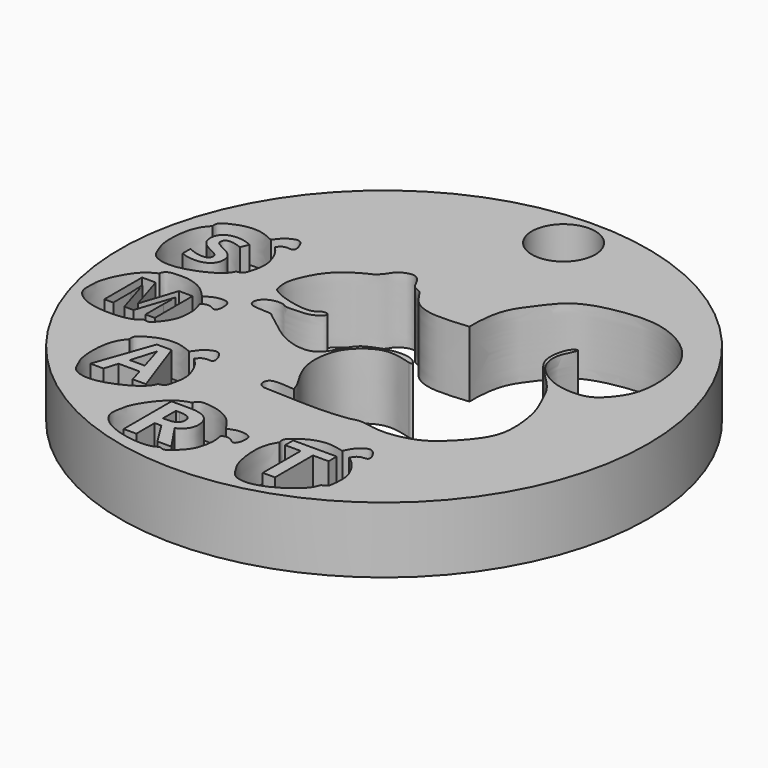
from build123d import *

# Parameters (mm, degrees)
F0_R           = 25.4
F1_DEPTH       = 6.35
F3_DEPTH       = 3.175
F4_TEXT_SIZE   = 6.6135069162
F4_TEXT_SIZE_2 = 6.365134491
F4_TEXT_SIZE_3 = 7.739350031
F4_TEXT_SIZE_4 = 8.0579310345
F4_TEXT_SIZE_5 = 7.7680943327
F5_DEPTH       = 3.175
F6_R           = 3.048
F7_DEPTH       = 25.4


# Not quite as in the source:
# - Text() gives the source's letters only with a copy of the font that has no kerning and outlines rounded to 1/6400 em; it was checked with that copy


with BuildPart() as f1:
    # F0 (on Top) → F1 (new body)
    with BuildSketch(Plane.XY):
        Circle(F0_R)
        with BuildLine():
            add(Edge.make_bspline(
                [(3.103984287, -0.8738507167), (3.2322647315, -0.8978823469), (3.5149160662, -0.9508333041), (3.1489052737, -0.3935869069), (2.1759216009, 0.01042191), (0.4678924032, -0.1717785151), (-0.6658792375, -0.6737219093), (-1.7045465622, -1.1078755571), (-2.5695800826, -2.8283012682), (-3.3167997934, -3.978649584), (-5.0026669085, -4.2655482317), (-7.292063398, -3.3539291003), (-8.8308556716, -1.9327427837), (-9.7776344556, -1.3804225536), (-9.9096110556, -1.0268847401), (-11.7269123051, -1.1581922681), (-12.2987806359, -0.6742192075), (-12.186278121, 0.0905562062), (-11.3044733094, 0.7354376931), (-10.1770359316, 0.7119397356), (-9.9059421857, 0.3673581843), (-8.4562468827, 0.44879459), (-7.5199595832, 0.5096907301), (-6.5266853491, 1.092838295), (-6.594417206, 1.6640416494), (-7.4144486566, 1.4846144189), (-7.7096041895, 1.0548830834), (-8.9475055661, 1.0261015402), (-10.6206031717, 1.4261002308), (-11.5516225248, 1.8097186625), (-11.9262345749, 2.0845401136), (-12.0926881209, 2.2066531237)],
                knots=[0, 0, 0, 0, 0.0184086765, 0.04056142, 0.0760871843, 0.1209751136, 0.1592656487, 0.1947406005, 0.2417782506, 0.2813138073, 0.3236254209, 0.3775272699, 0.42833216, 0.4622779251, 0.4810085106, 0.5258803693, 0.5538009145, 0.5810631125, 0.6164897777, 0.6512938544, 0.6727879582, 0.7125289418, 0.7482314257, 0.7830455257, 0.8029526961, 0.8310756273, 0.8553552773, 0.8920195713, 0.9381311083, 0.9725094363, 1, 1, 1, 1], degree=3))
            add(Edge.make_bspline(
                [(-12.0926881209, 2.2066531237), (-12.1940696834, 2.6175798085), (-12.4176238462, 3.5237048342), (-11.7188787033, 5.3710118016), (-10.5601116678, 7.2426050922), (-8.4458315601, 8.4856568685), (-7.8733042, 8.650989017), (-7.19697809, 9.3700944594), (-6.9202423533, 10.0770039736), (-5.3336173542, 10.8016234373), (-4.5255374898, 9.5922548337), (-4.2877600091, 8.857299522), (-3.3906737996, 8.7893316439), (-2.7399658464, 7.2252450905), (-0.7680652696, 6.1582634822), (1.620715387, 6.3925439066), (2.9963927809, 6.5274639055)],
                knots=[0, 0, 0, 0, 0.0677915818, 0.1494856652, 0.2403248537, 0.3309571532, 0.3772706487, 0.4332906216, 0.4864872395, 0.5575025948, 0.6239020411, 0.6741953722, 0.7244037027, 0.7978595843, 0.8835891443, 1, 1, 1, 1], degree=3))
            add(Edge.make_bspline(
                [(2.9963927809, 6.5274639055), (2.9876517934, 6.8087234454), (2.9646580281, 7.5485958891), (3.2208507353, 10.2567825473), (4.8072550972, 12.248326722), (6.4649635254, 14.6254966411), (10.2089734272, 15.6611927232), (14.460945516, 15.9289527113), (18.5488481139, 13.4786584252), (19.8526536032, 9.7353067267), (19.8012884144, 6.002184071), (18.3256681545, 4.0448117291), (17.1799807769, 3.0665154622), (15.2183525329, 2.921829898), (13.2866030879, 3.370569802), (11.2108415273, 4.8912140214), (10.9518605827, 6.9579767834), (11.7126375257, 8.1676137563), (11.835203024, 8.7609334617), (11.0376890387, 8.3226443822), (10.6454263926, 6.4262151181), (11.1367654893, 4.8472956079), (13.8780378076, 2.639052327), (14.6193307744, 0.6775555704), (15.5764121145, -1.0553911706), (16.0893294875, -4.7364792027), (15.2584275057, -6.994987292), (13.0169948018, -9.4077268957), (11.3436454874, -10.4962327281), (8.3671834629, -11.1056107936), (6.2922127831, -10.4818220399), (5.4045318163, -10.8220613007), (2.7361227002, -11.1025647871), (-0.7484432709, -10.9461593333), (-2.863347996, -10.8512314036)],
                knots=[0, 0, 0, 0, 0.0202729676, 0.053329427, 0.0862177936, 0.1201814784, 0.1596746732, 0.2019328198, 0.2448843541, 0.2850521519, 0.3240146713, 0.3551185648, 0.3795745039, 0.4073235043, 0.4364616357, 0.4683388439, 0.4966906712, 0.5211328686, 0.5330672025, 0.5484253259, 0.576298053, 0.6025702825, 0.64030066, 0.669735875, 0.6984825795, 0.7371358216, 0.7691791352, 0.8054178117, 0.8347329346, 0.8700946245, 0.8994017724, 0.9182660249, 0.9503927974, 1, 1, 1, 1], degree=3))
            add(Edge.make_bspline(
                [(-2.863347996, -10.8512314036), (-3.061201015, -10.7826228229), (-3.4528073756, -10.6468272878), (-3.4972516428, -9.9779984455), (-3.0791354632, -9.4406366165), (-1.8051631092, -9.5707881165), (-0.9538021986, -9.6577648073)],
                knots=[0, 0, 0, 0, 0.2061926485, 0.4081128157, 0.6044579691, 1, 1, 1, 1], degree=3))
            add(Edge.make_bspline(
                [(-0.9538021986, -9.6577648073), (-1.0367983248, -9.4054360401), (-1.2309611872, -8.8151328783), (-2.1203573849, -7.5419054583), (-2.8889914343, -5.566129078), (-2.5841219867, -3.1496157847), (-1.6860903105, -1.6892751952), (0.4167129584, -0.1296739464), (2.1877894843, -0.6201320535), (3.103984287, -0.8738507167)],
                knots=[0, 0, 0, 0, 0.0956691445, 0.2238103847, 0.3757763894, 0.5344064878, 0.6700913312, 0.8293350946, 1, 1, 1, 1], degree=3))
        make_face(mode=Mode.SUBTRACT)
    extrude(amount=F1_DEPTH)

    # F2 (on face) → F3 (cut)
    with BuildSketch(Plane.XY.offset(6.35)):
        with BuildLine():
            add(Edge.make_bspline(
                [(-15.7901886851, -2.1640327759), (-15.6233715735, -2.0610756288), (-15.2793392474, -1.8487437736), (-14.67686474, -1.6057684903), (-13.8798895675, -1.5693358789), (-13.5422659371, -1.8656144949), (-13.4470080058, -2.264291287), (-13.4364409048, -2.7678864415), (-13.5653795033, -3.2291524635), (-13.8678948177, -3.2838129775), (-14.1769044709, -3.0379750783), (-14.7016816147, -2.9581138498), (-15.0024854487, -3.1334746955), (-15.153802, -3.2216883264)],
                knots=[0, 0, 0, 0, 0.1008453758, 0.2079766811, 0.3225392504, 0.4051553152, 0.4869615092, 0.5820025773, 0.6686043419, 0.7322039204, 0.8129866828, 0.9059247024, 1, 1, 1, 1], degree=3))
            add(Edge.make_bspline(
                [(-20.6172689795, -1.2725904817), (-20.6087974536, -1.2117912647), (-20.5891104199, -1.0704995726), (-20.3953294443, -0.7396335329), (-19.8462206021, -0.577487435), (-18.9891890187, -0.555969218), (-18.2456609338, -0.5948161099), (-17.3589451487, -0.8670013599), (-16.5927339426, -1.3128013551), (-16.0700836546, -1.8671580634), (-15.7901886851, -2.1640327759)],
                knots=[0, 0, 0, 0, 0.0677876766, 0.1575322185, 0.2708871515, 0.4126239652, 0.5459218156, 0.6908263252, 0.834428186, 1, 1, 1, 1], degree=3))
            add(Edge.make_bspline(
                [(-16.809143126, -7.864783518), (-16.9774106863, -8.0003104644), (-17.3400812084, -8.2924144704), (-18.2138042015, -8.5410084944), (-19.3016097501, -8.6358970413), (-20.5889961529, -8.6094652324), (-22.1926803585, -8.2654948905), (-23.3026210763, -7.380002413), (-23.4768975603, -6.6082471653), (-23.4360958252, -6.0359384407), (-23.465265648, -5.3628975781), (-23.1878528901, -4.3403679544), (-22.6188328687, -3.1304425293), (-22.037375349, -2.2801874143), (-21.3409424037, -1.6086884742), (-20.8512880477, -1.3812767155), (-20.6172689795, -1.2725904817)],
                knots=[0, 0, 0, 0, 0.0587483623, 0.1266215496, 0.2018658275, 0.2840303707, 0.3768702365, 0.4607027922, 0.5222865729, 0.5760184143, 0.6342303199, 0.7084450361, 0.7923621537, 0.866042282, 0.9359779813, 1, 1, 1, 1], degree=3))
            add(Edge.make_bspline(
                [(-15.153802, -3.2216883264), (-15.1125022344, -3.3265279303), (-15.0103246606, -3.5859060694), (-14.7903293322, -4.3698597248), (-14.8318392985, -5.5472467776), (-15.0607052732, -6.4936040818), (-15.9114591906, -7.6293387712), (-16.3019229336, -7.9872551144), (-16.6402077563, -7.9055740558), (-16.809143126, -7.864783518)],
                knots=[0, 0, 0, 0, 0.0987604967, 0.2443381403, 0.4196982307, 0.5836796249, 0.7750862549, 0.8876807822, 1, 1, 1, 1], degree=3))
        make_face()
        with BuildLine():
            add(Edge.make_bspline(
                [(-10.9250828015, -9.7823362647), (-10.8174067247, -9.6185254428), (-10.5953428682, -9.2806930853), (-10.1520013225, -8.805865965), (-9.4450936045, -8.4360305435), (-9.0138899255, -8.5618642485), (-8.7590688277, -8.8829303883), (-8.536663273, -9.3348767485), (-8.4585818844, -9.8074175425), (-8.7096533381, -9.9848052884), (-9.0936067788, -9.8925936084), (-9.6029672042, -10.0419951595), (-9.8014773656, -10.3280512529), (-9.9013360429, -10.4719490915)],
                knots=[0, 0, 0, 0, 0.1008453758, 0.2079766811, 0.3225392504, 0.4051553152, 0.4869615092, 0.5820025773, 0.6686043419, 0.7322039204, 0.8129866828, 0.9059247024, 1, 1, 1, 1], degree=3))
            add(Edge.make_bspline(
                [(-15.6766430538, -11.0144274551), (-15.6946601033, -10.9557444297), (-15.7365300407, -10.8193705689), (-15.7007348641, -10.4376087216), (-15.2715991465, -10.0585910261), (-14.5039587402, -9.6768917004), (-13.813676041, -9.3978703942), (-12.8950081629, -9.269811722), (-12.0121817612, -9.3500288811), (-11.3042184669, -9.6315651265), (-10.9250828015, -9.7823362647)],
                knots=[0, 0, 0, 0, 0.0677876766, 0.1575322185, 0.2708871515, 0.4126239652, 0.5459218156, 0.6908263252, 0.834428186, 1, 1, 1, 1], degree=3))
            add(Edge.make_bspline(
                [(-9.4393277767, -15.3795998088), (-9.5345538143, -15.5735418795), (-9.7397964454, -15.9915492004), (-10.4265980235, -16.5861031928), (-11.3723830302, -17.1318279117), (-12.5503219171, -17.6519455613), (-14.1491215486, -18.0179487932), (-15.5292947559, -17.6845012824), (-16.0134007518, -17.0587059164), (-16.2182899399, -16.5227745043), (-16.5291661368, -15.9251200293), (-16.7098844862, -14.8811537714), (-16.7055137899, -13.5441106846), (-16.5378676508, -12.5277832866), (-16.1904727641, -11.6248732875), (-15.8428035704, -11.2118313669), (-15.6766430538, -11.0144274551)],
                knots=[0, 0, 0, 0, 0.0587483623, 0.1266215496, 0.2018658275, 0.2840303707, 0.3768702365, 0.4607027922, 0.5222865729, 0.5760184143, 0.6342303199, 0.7084450361, 0.7923621537, 0.866042282, 0.9359779813, 1, 1, 1, 1], degree=3))
            add(Edge.make_bspline(
                [(-9.9013360429, -10.4719490915), (-9.8195986126, -10.5495120057), (-9.6173763436, -10.7414063243), (-9.0866797332, -11.3589355836), (-8.6267152692, -12.4435535077), (-8.4341904054, -13.3979674423), (-8.7252530854, -14.786836777), (-8.9278714334, -15.2762362543), (-9.2689815094, -15.3451734185), (-9.4393277767, -15.3795998088)],
                knots=[0, 0, 0, 0, 0.0987604967, 0.2443381403, 0.4196982307, 0.5836796248, 0.7750862549, 0.8876807822, 1, 1, 1, 1], degree=3))
        make_face()
        with BuildLine():
            add(Edge.make_bspline(
                [(-0.9390761488, -17.8601125691), (-0.756915043, -17.7876870598), (-0.3812383013, -17.638321589), (0.2542754798, -17.5036562467), (1.0454692652, -17.6061704148), (1.3265153922, -17.956575621), (1.3510966431, -18.365736983), (1.2740548253, -18.8635163534), (1.0669770896, -19.2953847554), (0.759565964, -19.2966836203), (0.4979401649, -19.000921588), (-0.0049966781, -18.8311470363), (-0.3316817173, -18.9516097191), (-0.4960175664, -19.0122073434)],
                knots=[0, 0, 0, 0, 0.1008453758, 0.2079766811, 0.3225392504, 0.4051553152, 0.4869615092, 0.5820025773, 0.6686043419, 0.7322039204, 0.8129866828, 0.9059247024, 1, 1, 1, 1], degree=3))
            add(Edge.make_bspline(
                [(-5.5380249174, -16.1439995898), (-5.5191244197, -16.0855951146), (-5.4752014314, -15.9498685782), (-5.2269101394, -15.6576788504), (-4.65798712, -15.5933478659), (-3.8102391728, -15.7209785316), (-3.0847526423, -15.888347549), (-2.258772535, -16.3103742735), (-1.5816141556, -16.8824527448), (-1.163167132, -17.5191447991), (-0.9390761488, -17.8601125691)],
                knots=[0, 0, 0, 0, 0.0677876766, 0.1575322185, 0.2708871515, 0.4126239652, 0.5459218156, 0.6908263252, 0.834428186, 1, 1, 1, 1], degree=3))
            add(Edge.make_bspline(
                [(-2.9324753599, -23.2973165161), (-3.1217205651, -23.4015651485), (-3.5296046354, -23.6262543629), (-4.4332217123, -23.7193512796), (-5.5209782735, -23.6239028051), (-6.7842165487, -23.374320252), (-8.3038073647, -22.7570987526), (-9.2431214339, -21.6923197126), (-9.2807363742, -20.9020263674), (-9.1411741421, -20.3454974452), (-9.0530284903, -19.677616299), (-8.6022698498, -18.7187934179), (-7.831793176, -17.6260587684), (-7.1115240513, -16.8896899777), (-6.3090669201, -16.3493269273), (-5.7873618765, -16.2103976508), (-5.5380249174, -16.1439995898)],
                knots=[0, 0, 0, 0, 0.0587483623, 0.1266215496, 0.2018658275, 0.2840303707, 0.3768702365, 0.4607027922, 0.5222865729, 0.5760184143, 0.6342303199, 0.7084450361, 0.7923621537, 0.866042282, 0.9359779813, 1, 1, 1, 1], degree=3))
            add(Edge.make_bspline(
                [(-0.4960175664, -19.0122073434), (-0.4735504432, -19.1226258272), (-0.4179657175, -19.395806379), (-0.3374447361, -20.2060518047), (-0.5827751889, -21.3583435726), (-0.9724973965, -22.2505814235), (-2.0075447094, -23.2213298835), (-2.4542279515, -23.5060053559), (-2.7731897006, -23.3668226731), (-2.9324753599, -23.2973165161)],
                knots=[0, 0, 0, 0, 0.0987604967, 0.2443381403, 0.4196982307, 0.5836796248, 0.7750862549, 0.8876807822, 1, 1, 1, 1], degree=3))
        make_face()
        with BuildLine():
            add(Edge.make_bspline(
                [(8.1548618025, -15.2248200443), (8.2394381631, -15.0479727597), (8.4138627279, -14.6832548833), (8.7890454501, -14.1529243776), (9.4395552573, -13.6910437096), (9.8837989038, -13.7575141284), (10.179630466, -14.0412410127), (10.4610117149, -14.4590260484), (10.6021701449, -14.9167003899), (10.3773439064, -15.126358325), (9.9844568547, -15.0868234916), (9.4999279708, -15.3036197718), (9.3418518257, -15.6138556581), (9.2623331015, -15.7699169149)],
                knots=[0, 0, 0, 0, 0.1008453758, 0.2079766811, 0.3225392504, 0.4051553152, 0.4869615092, 0.5820025773, 0.6686043419, 0.7322039204, 0.8129866828, 0.9059247024, 1, 1, 1, 1], degree=3))
            add(Edge.make_bspline(
                [(3.6131267607, -17.0870811278), (3.5873525814, -17.0313675458), (3.5274558001, -16.9018943936), (3.5113864294, -16.5187949574), (3.8854273925, -16.0853145823), (4.5945123409, -15.6034798547), (5.2408089896, -15.2338263199), (6.1337797378, -14.9829220818), (7.0193538107, -14.9432256147), (7.7588430462, -15.1266114217), (8.1548618025, -15.2248200443)],
                knots=[0, 0, 0, 0, 0.0677876766, 0.1575322185, 0.2708871515, 0.4126239652, 0.5459218156, 0.6908263252, 0.834428186, 1, 1, 1, 1], degree=3))
            add(Edge.make_bspline(
                [(10.3826324567, -20.570272793), (10.3144598085, -20.7752947799), (10.1675259025, -21.2171828711), (9.5672746168, -21.8990107464), (8.7038188234, -22.5674184368), (7.6068774099, -23.2417936485), (6.0721227804, -23.820280342), (4.6595691895, -23.6762050928), (4.0954139469, -23.1214913671), (3.8200509509, -22.6181254184), (3.4313387008, -22.0679093991), (3.1113418731, -21.0578961815), (2.9351751511, -19.7325024267), (2.9640850403, -18.7028467434), (3.1864093069, -17.7613046072), (3.4751363114, -17.3051092398), (3.6131267607, -17.0870811278)],
                knots=[0, 0, 0, 0, 0.0587483623, 0.1266215496, 0.2018658275, 0.2840303707, 0.3768702365, 0.4607027922, 0.5222865729, 0.5760184143, 0.6342303199, 0.7084450361, 0.7923621537, 0.866042282, 0.9359779813, 1, 1, 1, 1], degree=3))
            add(Edge.make_bspline(
                [(9.2623331015, -15.7699169149), (9.3537930987, -15.8357354693), (9.580069458, -15.998573686), (10.1892729188, -16.5388073593), (10.7914474982, -17.5514026018), (11.1110534275, -18.4710894136), (11.0101489711, -19.8865376829), (10.8754530845, -20.3988101314), (10.54677189, -20.5131652319), (10.3826324567, -20.570272793)],
                knots=[0, 0, 0, 0, 0.0987604967, 0.2443381403, 0.4196982307, 0.5836796248, 0.7750862549, 0.8876807822, 1, 1, 1, 1], degree=3))
        make_face()
        with BuildLine():
            add(Edge.make_bspline(
                [(-17.5004055036, 8.2499598389), (-17.3848422249, 8.408305194), (-17.1465123368, 8.7348659426), (-16.6804659243, 9.1874289347), (-15.9563069583, 9.5222282069), (-15.531777659, 9.375443984), (-15.2929734677, 9.0422926426), (-15.0929507052, 8.5800041637), (-15.0380870022, 8.104208536), (-15.2975382569, 7.9393196835), (-15.6765192461, 8.0502099371), (-16.1925804983, 7.9259133146), (-16.4048512, 7.6499141806), (-16.5116319883, 7.5110754013)],
                knots=[0, 0, 0, 0, 0.1008453758, 0.2079766811, 0.3225392504, 0.4051553152, 0.4869615092, 0.5820025773, 0.6686043419, 0.7322039204, 0.8129866828, 0.9059247024, 1, 1, 1, 1], degree=3))
            add(Edge.make_bspline(
                [(-22.3065663543, 7.2518659502), (-22.3216901201, 7.311360347), (-22.356836337, 7.4496197589), (-22.302402243, 7.8291725644), (-21.8552331453, 8.1867360911), (-21.0698336839, 8.5304130541), (-20.3667238758, 8.7753205706), (-19.4428899802, 8.858270117), (-18.5650467546, 8.734947291), (-17.8717088385, 8.4191036309), (-17.5004055036, 8.2499598389)],
                knots=[0, 0, 0, 0, 0.0677876766, 0.1575322185, 0.2708871515, 0.4126239652, 0.5459218156, 0.6908263252, 0.834428186, 1, 1, 1, 1], degree=3))
            add(Edge.make_bspline(
                [(-16.2903368135, 2.5866956792), (-16.3949394644, 2.3976459227), (-16.6203917022, 1.9901831067), (-17.3354653889, 1.4299505834), (-18.3068227263, 0.9311623811), (-19.5088027058, 0.4693111935), (-21.1235975039, 0.1819849199), (-22.4857996607, 0.582572749), (-22.9387018968, 1.2313084576), (-23.1171194071, 1.7766241918), (-23.3983764816, 2.3887755941), (-23.5277910449, 3.4403346938), (-23.4579963777, 4.7755620241), (-23.2408163463, 5.7824678995), (-22.8496530849, 6.6672961182), (-22.4821879073, 7.062829732), (-22.3065663543, 7.2518659502)],
                knots=[0, 0, 0, 0, 0.0587483623, 0.1266215496, 0.2018658275, 0.2840303707, 0.3768702365, 0.4607027922, 0.5222865729, 0.5760184143, 0.6342303199, 0.7084450361, 0.7923621537, 0.866042282, 0.9359779813, 1, 1, 1, 1], degree=3))
            add(Edge.make_bspline(
                [(-16.5116319883, 7.5110754013), (-16.4337880847, 7.4296055305), (-16.241198585, 7.2280452164), (-15.741357045, 6.5852857643), (-15.3350202438, 5.4794585837), (-15.189431001, 4.5167667566), (-15.5481103307, 3.1438047574), (-15.7744350583, 2.6649068967), (-16.118509952, 2.6127448018), (-16.2903368135, 2.5866956792)],
                knots=[0, 0, 0, 0, 0.0987604967, 0.2443381403, 0.4196982307, 0.5836796248, 0.7750862549, 0.8876807822, 1, 1, 1, 1], degree=3))
        make_face()
    extrude(amount=-F3_DEPTH, mode=Mode.SUBTRACT)

    # F4 (on face) → F5 (join)
    with BuildSketch(Plane.XY.offset(3.175)):
        with Locations((-21.59, 2.1669884748)):
            Text('S', F4_TEXT_SIZE, font='Open Sans', font_style=FontStyle.BOLD, text_align=(TextAlign.LEFT, TextAlign.BOTTOM))
        with Locations((-21.7881663287, -7.1326487281)):
            Text('M', F4_TEXT_SIZE_2, font='Open Sans', font_style=FontStyle.BOLD, text_align=(TextAlign.LEFT, TextAlign.BOTTOM))
        with Locations((-15.494, -15.9644959025)):
            Text('A', F4_TEXT_SIZE_3, font='Open Sans', font_style=FontStyle.BOLD, text_align=(TextAlign.LEFT, TextAlign.BOTTOM))
        with Locations((-7.62, -22.7080127671)):
            Text('R', F4_TEXT_SIZE_4, font='Open Sans', font_style=FontStyle.BOLD, text_align=(TextAlign.LEFT, TextAlign.BOTTOM))
        with Locations((4.064, -21.75289765)):
            Text('T', F4_TEXT_SIZE_5, font='Open Sans', font_style=FontStyle.BOLD, text_align=(TextAlign.LEFT, TextAlign.BOTTOM))
    extrude(amount=F5_DEPTH)

    # F6 (on face) → F7 (cut)
    with BuildSketch(Plane.XY.offset(6.35)):
        with Locations((0, 21.59)):
            Circle(F6_R)
    extrude(amount=-F7_DEPTH, mode=Mode.SUBTRACT)


solid = f1.part
